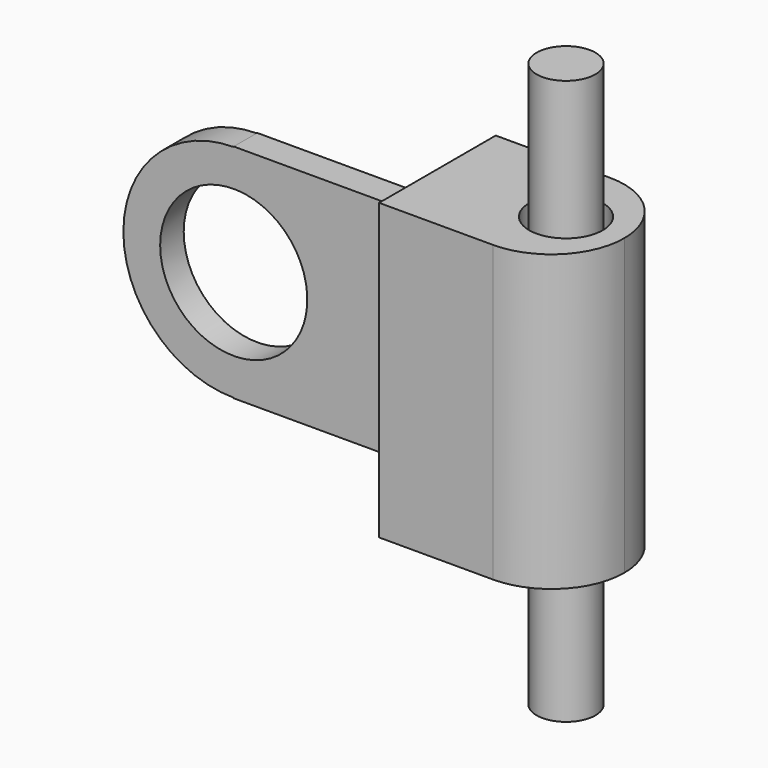
from build123d import *

# Parameters (mm, degrees)
F0_R      = 15
F1_DEPTH  = 2
F3_W      = 26.0858
F3_H      = 15.0651354343
F4_DEPTH  = 2
F6_D      = 20
F7_W      = 19.812
F7_H      = 40.0436846481
F7_W_2    = 4
F7_H_2    = 30.1302708685
F8_DEPTH  = 25.4
F9_R      = 9.90599
F11_D     = 10
F12_R     = 4
F13_DEPTH = 38.354


# Not quite as in the source:
# - a fillet or chamfer is up to 0.001 mm smaller than in the source, because OpenCascade refuses the exact size


with BuildPart() as f1:
    # F0 (on Front) → F1 (new body, symmetric)
    with BuildSketch(Plane.XZ):
        Circle(F0_R)
    extrude(amount=F1_DEPTH, both=True)

    # F3 (on Front) → F4 (join, symmetric)
    with BuildSketch(Plane.XZ):
        with Locations((13.0429, 7.5325677171)):
            Rectangle(F3_W, F3_H)
    extrude(amount=F4_DEPTH, both=True)

    # F5: F1 across plane


with BuildPart() as f1_1:
    add(f1.part)
    add(f1.part.mirror(Plane.XY))

    # F6 (through all)
    with Locations(Plane.XZ.offset(2)):
        with Locations((0, 0)):
            Hole(F6_D / 2)


with BuildPart() as f8:
    # F7 (on face) → F8 (new body)
    with BuildSketch(Plane.YZ.offset(26.0858)):
        Rectangle(F7_W, F7_H)
        Rectangle(F7_W_2, F7_H_2, mode=Mode.SUBTRACT)
        Rectangle(F7_W_2, F7_H_2)
    extrude(amount=F8_DEPTH)

    # F9 (radius 9.906 in the source; OpenCascade refuses exactly that, so slightly less here)
    f9_edges = [f8.edges().sort_by_distance(p)[0] for p in [
        (51.4858, -9.906, 0),
        (51.4858, 9.906, 0),
    ]]
    fillet(f9_edges, radius=F9_R)

    # F11 (through all)
    with Locations(Plane(origin=(0, 0, -20.021842324), x_dir=(1, 0, 0), z_dir=(0, 0, -1))):
        with Locations((43.5614921153, 0)):
            Hole(F11_D / 2)


with BuildPart() as f13:
    # F12 (on Top) → F13 (new body, symmetric)
    with BuildSketch(Plane.XY):
        with Locations((43.5654483736, 0)):
            Circle(F12_R)
    extrude(amount=F13_DEPTH, both=True)


solid = Compound([f1_1.part, f8.part, f13.part])
